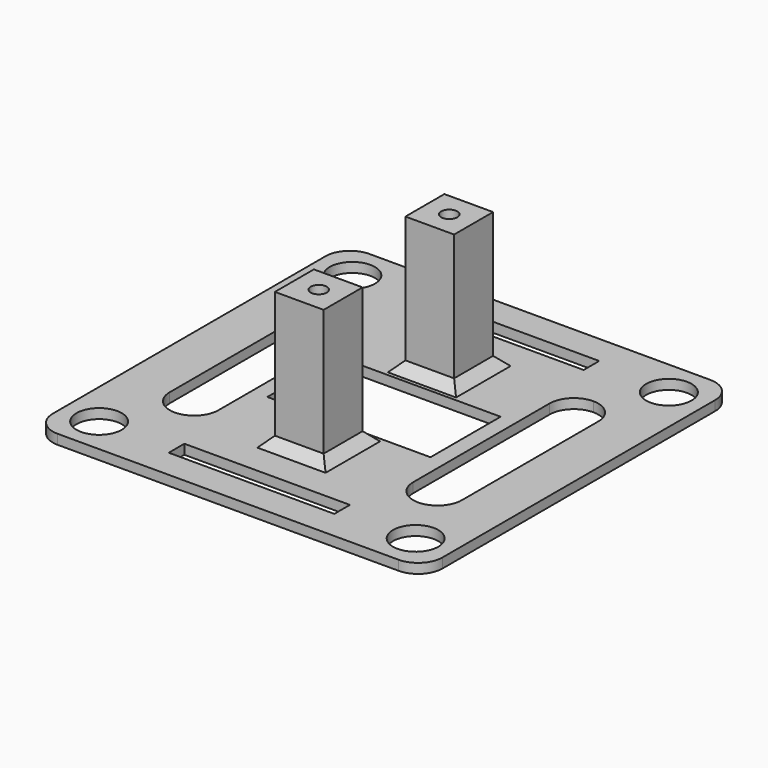
from build123d import *

# Parameters (mm, degrees)
F0_W     = 10
F0_H     = 10
F0_R     = 1.65
F1_DEPTH = 30
F0_W_2   = 80
F0_H_2   = 80
F0_R_2   = 4.65
F0_W_3   = 33.5
F0_H_3   = 18.0101236328
F2_DEPTH = 2
F3_R     = 5
F4_SIZE  = 2
F5_W     = 34
F5_H     = 4
F6_DEPTH = 25


with BuildPart() as f1:
    # F0 (on Top) → F1 (new body)
    with BuildSketch(Plane.XY):
        with Locations((-0.4196270893, 17.7291296907)):
            Rectangle(F0_W, F0_H)
        with Locations((-0.4196270893, 17.7291296907)):
            Circle(F0_R, mode=Mode.SUBTRACT)
    extrude(amount=F1_DEPTH)



with BuildPart() as f1b:
    # F0 (on Top) → F1, piece 2 (new body)
    with BuildSketch(Plane.XY):
        with Locations((-0.4196270893, -15.7708703093)):
            Rectangle(F0_W, F0_H)
        with Locations((-0.4196270893, -15.7708703093)):
            Circle(F0_R, mode=Mode.SUBTRACT)
    extrude(amount=F1_DEPTH)


with BuildPart() as f1_1:
    add(f1.part)

    add(f1b.part)  # F2 merges F1b
    # F0 (on Top) → F2 (join)
    with BuildSketch(Plane.XY):
        with Locations((-0.4196270893, 0.9791296907)):
            Rectangle(F0_W_2, F0_H_2)
        with Locations((-32.9196270893, -31.5208703093)):
            Circle(F0_R_2, mode=Mode.SUBTRACT)
        with Locations((32.0803729107, -31.5208703093)):
            Circle(F0_R_2, mode=Mode.SUBTRACT)
        with Locations((-0.4196270893, -15.7708703093)):
            Rectangle(F0_W, F0_H, mode=Mode.SUBTRACT)
        with Locations((-32.9196270893, 33.4791296907)):
            Circle(F0_R_2, mode=Mode.SUBTRACT)
        with Locations((-0.4196270893, 0.9791296907)):
            Rectangle(F0_W_3, F0_H_3, mode=Mode.SUBTRACT)
        with Locations((-0.4196270893, 17.7291296907)):
            Rectangle(F0_W, F0_H, mode=Mode.SUBTRACT)
        with Locations((32.0803729107, 33.4791296907)):
            Circle(F0_R_2, mode=Mode.SUBTRACT)
    extrude(amount=F2_DEPTH)

    # F3
    f3_edges = [f1_1.edges().sort_by_distance(p)[0] for p in [
        (-40.419627, -39.02087, 1),
        (-40.419627, 40.97913, 1),
        (39.580373, -39.02087, 1),
        (39.580373, 40.97913, 1),
    ]]
    fillet(f3_edges, radius=F3_R)

    # F4
    f4_edges = [f1_1.edges().sort_by_distance(p)[0] for p in [
        (-0.419627, 22.72913, 2),
        (-0.419627, -10.77087, 2),
        (4.580373, -15.77087, 2),
        (4.580373, 17.72913, 2),
        (-0.419627, -20.77087, 2),
        (-0.419627, 12.72913, 2),
        (-5.419627, 17.72913, 2),
        (-5.419627, -15.77087, 2),
    ]]
    chamfer(f4_edges, length=F4_SIZE)

    # F5 (on face) → F6 (cut)
    with BuildSketch(Plane.XY.offset(2)):
        with BuildLine():
            Line((-20.4196270893, -16.5208703093), (-20.4196270893, 18.4791296907))
            ThreePointArc((-20.4196270893, 18.4791296907), (-21.8840931834, 22.0146635966), (-25.4196270893, 23.4791296907))
            ThreePointArc((-25.4196270893, 23.4791296907), (-28.9551609952, 22.0146635966), (-30.4196270893, 18.4791296907))
            Line((-30.4196270893, 18.4791296907), (-30.4196270893, -16.5208703093))
            ThreePointArc((-30.4196270893, -16.5208703093), (-28.9551609952, -20.0564042153), (-25.4196270893, -21.5208703093))
            ThreePointArc((-25.4196270893, -21.5208703093), (-21.8840931834, -20.0564042153), (-20.4196270893, -16.5208703093))
        make_face()
        with Locations((-0.4196270893, 32.9791296907)):
            Rectangle(F5_W, F5_H)
        with BuildLine():
            ThreePointArc((24.5803729107, 23.4791296907), (21.0448390048, 22.0146635966), (19.5803729107, 18.4791296907))
            Line((19.5803729107, 18.4791296907), (19.5803729107, -16.5208703093))
            ThreePointArc((19.5803729107, -16.5208703093), (21.0448390048, -20.0564042153), (24.5803729107, -21.5208703093))
            ThreePointArc((24.5803729107, -21.5208703093), (28.1159068166, -20.0564042153), (29.5803729107, -16.5208703093))
            Line((29.5803729107, -16.5208703093), (29.5803729107, 18.4791296907))
            ThreePointArc((29.5803729107, 18.4791296907), (28.1159068166, 22.0146635966), (24.5803729107, 23.4791296907))
        make_face()
        with Locations((-0.4196270893, -31.0208703093)):
            Rectangle(F5_W, F5_H)
    extrude(amount=-F6_DEPTH, mode=Mode.SUBTRACT)


solid = f1_1.part
